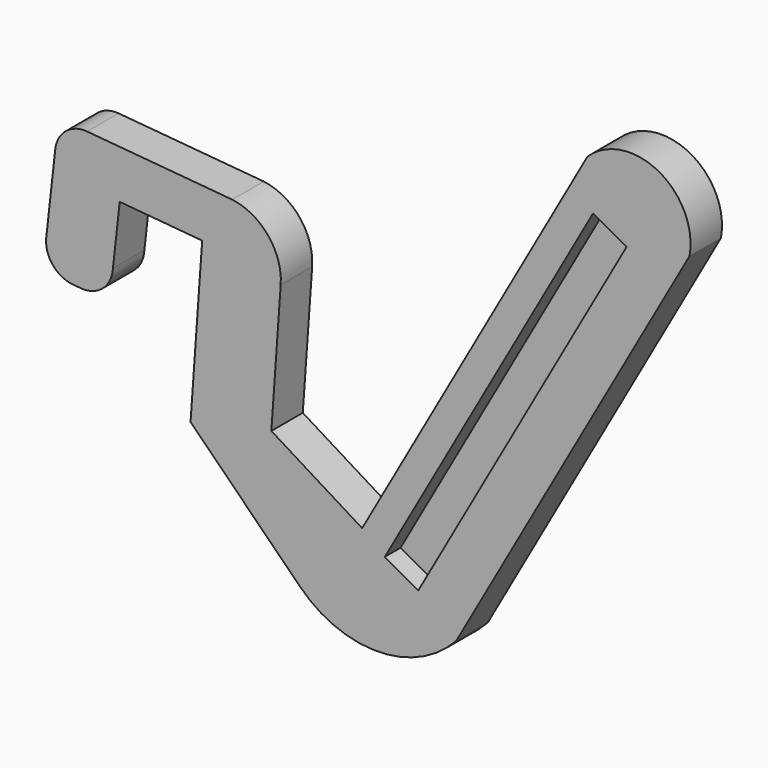
from build123d import *

# Parameters (mm, degrees)
F1_DEPTH = 4
F2_DEPTH = 2


# Not quite as in the source:
# - a feature names something its author has since deleted; it is built from what else it names


with BuildPart() as f1:
    # F0 (on Front) → F1 (new body)
    with BuildSketch(Plane.XZ):
        with BuildLine():
            ThreePointArc((-69.017292897, 29.3982457694), (-68.3268421331, 27.2084157133), (-66.290176034, 26.1481944472))
            Line((-66.290176034, 26.1481944472), (-65.4847666663, 26.0777302572))
            ThreePointArc((-65.4847666663, 26.0777302572), (-63.2535898646, 26.8035186892), (-62.2272009721, 28.913363378))
            Line((-62.2272009721, 28.913363378), (-61.5372568785, 35.1033145465))
            Line((-61.5372568785, 35.1033145465), (-53.1481667688, 34.3565562926))
            Line((-53.1481667688, 34.3565562926), (-54.3320948451, 17.7259296179))
            Line((-54.3320948451, 17.7259296179), (-43.1615771204, 6.577645293))
            ThreePointArc((-43.1615771204, 6.577645293), (-35.1559477392, 3.3688057895), (-27.2990026255, 6.9262158348))
            Line((-27.2990026255, 6.9262158348), (-3.5743886341, 49.0892314075))
            ThreePointArc((-3.5743886341, 49.0892314075), (-6.738115065, 55.6702900526), (-13.9632260986, 54.6132808892))
            Line((-13.9632260986, 54.6132808892), (-36.8751008064, 13.8946529478))
            Line((-36.8751008064, 13.8946529478), (-46.112828888, 19.5994470268))
            Line((-46.112828888, 19.5994470268), (-45.1602484403, 32.9947581421))
            ThreePointArc((-45.1602484403, 32.9947581421), (-46.4251891271, 36.9862585641), (-50.0833280385, 39.0234552324))
            Line((-50.0833280385, 39.0234552324), (-64.8513762012, 40.3222609912))
            ThreePointArc((-64.8513762012, 40.3222609912), (-67.0146267862, 39.6550864105), (-68.0957389782, 37.666124007))
            Line((-68.0957389782, 37.666124007), (-69.017292897, 29.3982457694))
        make_face()
        Polygon((-9.9778777986, 47.8288231225), (-31.1708185564, 10.1650579072), (-34.5696903843, 12.0775615796), (-13.3767496278, 49.7413267956), align=None, mode=Mode.SUBTRACT)
    extrude(amount=F1_DEPTH)

    # F0 (on Front) → F2 (join)
    with BuildSketch(Plane.XZ):
        Polygon((-34.5696903843, 12.0775615796), (-31.1708185564, 10.1650579072), (-9.9778777986, 47.8288231225), (-13.3767496278, 49.7413267956), align=None)
    extrude(amount=F2_DEPTH)


solid = f1.part
